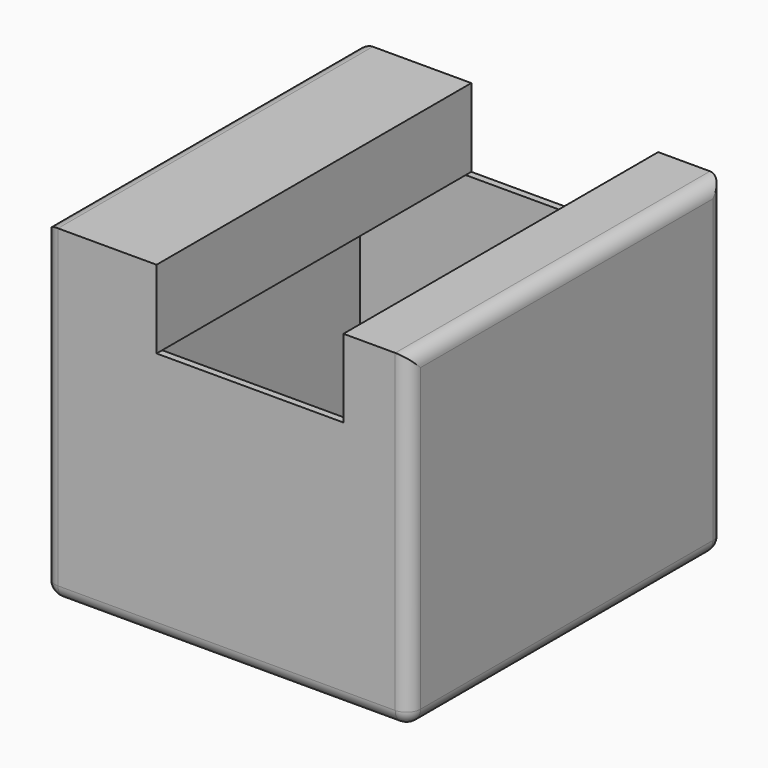
from build123d import *

# Parameters (mm, degrees)
F1_DEPTH = 140
F2_T     = -2.5
F3_R     = 5


# Not quite as in the source:
# - a shell that OpenCascade refuses in one call is made with other operations: the cavity is built on its own and cut out


with BuildPart() as f1:
    # F0 (on Front) → F1 (new body)
    with BuildSketch(Plane.XZ):
        Polygon((-68.4042458236, 42.9600325577), (-68.4042458236, -74.0399674423), (61.5957541764, -74.0399674423), (61.5957541764, 42.9600325577), (38.1572941835, 42.9600325577), (38.1572941835, 15.1600325577), (-28.3427058165, 15.1600325577), (-28.3427058165, 42.9600325577), align=None)
    extrude(amount=F1_DEPTH)

    # F2: a shell. OpenCascade refuses it in one call, so the cavity is built on its own and cut out:
    # the body offset inwards by the wall thickness, plus a prism from it out through each open face.
    f2_core = offset(f1.part, amount=F2_T, kind=Kind.INTERSECTION, mode=Mode.PRIVATE)
    f2_exits = [f2_core.faces().sort_by_distance(p)[0] for p in [
        (4.907294, -70, 12.660033),
    ]]
    add(f2_core, mode=Mode.SUBTRACT)
    extrude(f2_exits, amount=-F2_T, mode=Mode.SUBTRACT)

    # F3
    f3_edges = [f1.edges().sort_by_distance(p)[0] for p in [
        (-68.404246, -70, 42.960033),
        (-68.404246, -70, -74.039967),
        (-68.404246, 0, -15.539967),
        (-68.404246, -140, -15.539967),
        (61.595754, -70, -74.039967),
        (61.595754, -70, 42.960033),
        (61.595754, 0, -15.539967),
        (61.595754, -140, -15.539967),
        (-3.404246, 0, -74.039967),
        (-3.404246, -140, -74.039967),
    ]]
    fillet(f3_edges, radius=F3_R)


solid = f1.part
